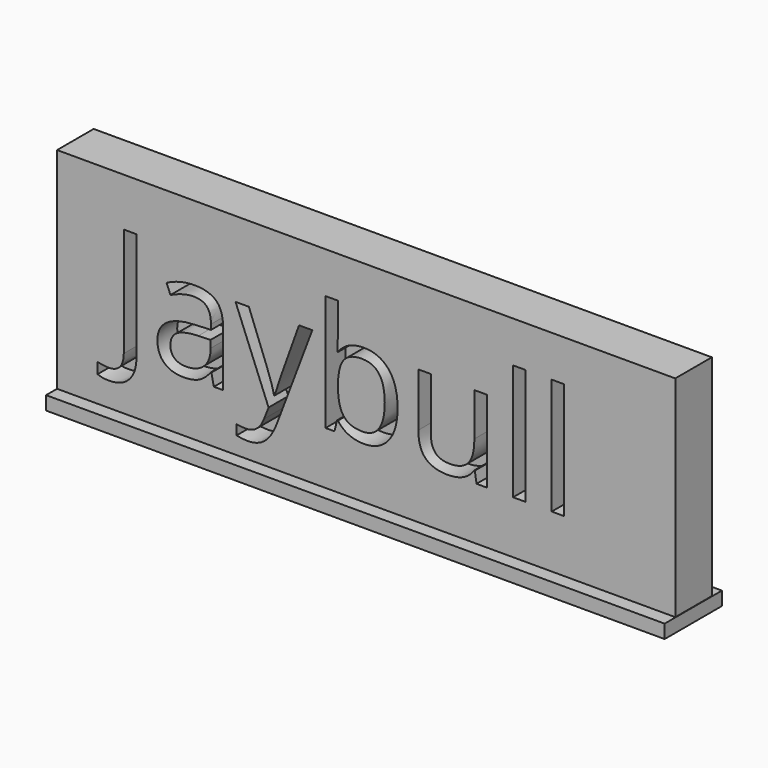
from build123d import *

# Parameters (mm, degrees)
F0_W         = 127
F0_H         = 43.18
F1_DEPTH     = 9.398
F2_TEXT_SIZE = 31.4028597333
F3_DEPTH     = 5.08
F4_W         = 127
F4_H         = 9.398
F5_DEPTH     = 2.794


# Not quite as in the source:
# - Text() gives the source's letters only with a copy of the font that has no kerning and outlines rounded to 1/6400 em; it was checked with that copy


with BuildPart() as f1:
    # F0 (on Front) → F1 (new body)
    with BuildSketch(Plane.XZ):
        with Locations((13.3405477811, 7.4183599158)):
            Rectangle(F0_W, F0_H)
    extrude(amount=F1_DEPTH)

    # F2 (on face) → F3 (cut)
    with BuildSketch(Plane.XZ.offset(9.398)):
        with Locations((-39.3706485629, -3.328303108)):
            Text('Jaybull', F2_TEXT_SIZE, font='Open Sans', text_align=(TextAlign.LEFT, TextAlign.BOTTOM))
    extrude(amount=-F3_DEPTH, mode=Mode.SUBTRACT)

    # F4 (on face) → F5 (join)
    with BuildSketch(Plane(origin=(0, 0, -14.1716400842), x_dir=(1, 0, 0), z_dir=(0, 0, -1))):
        Polygon((-50.1594522189, 0), (-50.1594522189, -2.4845025036), (76.9216120243, -2.4845025036), (76.9216120243, 12.2229540721), (-50.1594522189, 12.2229540721), (-50.1594522189, 9.398), (76.8405477811, 9.398), (76.8405477811, 0), align=None)
        with Locations((13.3405477811, 4.699)):
            Rectangle(F4_W, F4_H)
    extrude(amount=F5_DEPTH)


solid = f1.part
